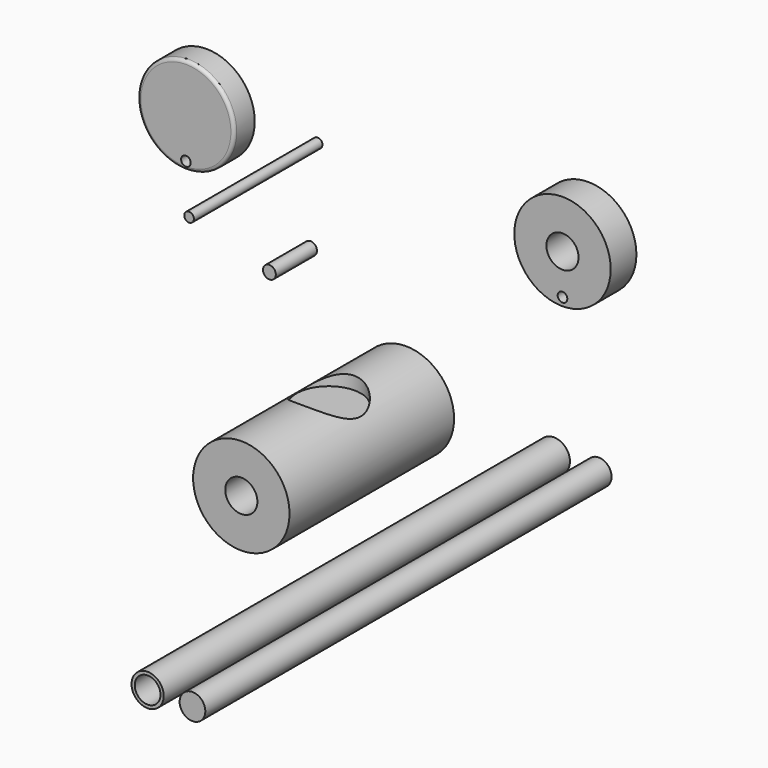
from build123d import *

# Parameters (mm, degrees)
F0_R      = 15
F0_R_2    = 5
F1_DEPTH  = 64
F2_R      = 2
F2_R_2    = 5
F3_DEPTH  = 3
F4_R      = 15
F4_R_2    = 2
F4_R_3    = 5
F5_DEPTH  = 10
F6_R      = 15
F6_R_2    = 1.5
F6_R_3    = 5
F7_DEPTH  = 2
F9_R      = 10
F10_DEPTH = 4
F11_R     = 5
F11_R_2   = 4
F12_DEPTH = 158
F13_R     = 4
F14_DEPTH = 158
F15_R     = 2
F16_DEPTH = 16
F17_R     = 15
F17_R_2   = 1.5
F18_DEPTH = 8
F19_R     = 1.5
F20_DEPTH = 50
F21_R     = 0.99999
F17_R_3   = 5
F22_DEPTH = 10
F23_R     = 5
F24_DEPTH = 5


# Not quite as in the source:
# - a fillet or chamfer is up to 0.001 mm smaller than in the source, because OpenCascade refuses the exact size
# - a feature names something its author has since deleted; it is built from what else it names


with BuildPart() as f1:
    # F0 (on Front) → F1 (new body)
    with BuildSketch(Plane.XZ):
        Circle(F0_R)
        Circle(F0_R_2, mode=Mode.SUBTRACT)
    extrude(amount=F1_DEPTH)

    # F9 (on offset) → F10 (cut)
    with BuildSketch(Plane.XY.offset(15)):
        with Locations((0, -30)):
            Circle(F9_R)
    extrude(amount=-F10_DEPTH, mode=Mode.SUBTRACT)


with BuildPart() as f3:
    # F2 (on Front) → F3 (new body)
    with BuildSketch(Plane.XZ):
        with BuildLine():
            Line((-54.3058665821, 6.5412230759), (-51.4285073808, 3.7625895941))
            ThreePointArc((-51.4285073808, 3.7625895941), (-48.3108465674, 8.5633662497), (-47.2186043859, 14.182465151))
            ThreePointArc((-47.2186043859, 14.182465151), (-67.8377032871, 28.0902229695), (-73.0087013909, 3.7625895941))
            Line((-73.0087013909, 3.7625895941), (-70.1313421896, 6.5412230759))
            ThreePointArc((-70.1313421896, 6.5412230759), (-62.2186043859, 3.182465151), (-54.3058665821, 6.5412230759))
        make_face()
        with Locations((-72.2186043859, 14.182465151)):
            Circle(F2_R, mode=Mode.SUBTRACT)
        with Locations((-62.2186043859, 14.182465151)):
            Circle(F2_R_2, mode=Mode.SUBTRACT)
        with BuildLine():
            ThreePointArc((-54.2186043859, 14.182465151), (-52.2186043859, 16.182465151), (-50.2186043859, 14.182465151))
            ThreePointArc((-50.2186043859, 14.182465151), (-52.2186043859, 12.182465151), (-54.2186043859, 14.182465151))
        make_face(mode=Mode.SUBTRACT)
    extrude(amount=F3_DEPTH)


with BuildPart() as f5:
    # F4 (on Front) → F5 (new body)
    with BuildSketch(Plane.XZ):
        with Locations((-47.7725118399, -37.5088863075)):
            Circle(F4_R)
        with Locations((-57.7725118399, -37.5088863075)):
            Circle(F4_R_2, mode=Mode.SUBTRACT)
        with Locations((-47.7725118399, -37.5088863075)):
            Circle(F4_R_3, mode=Mode.SUBTRACT)
        with Locations((-37.7725118399, -37.5088863075)):
            Circle(F4_R_2, mode=Mode.SUBTRACT)
    extrude(amount=F5_DEPTH)


with BuildPart() as f7:
    # F6 (on Front) → F7 (new body)
    with BuildSketch(Plane.XZ):
        with Locations((12.6999374479, 49.0343069208)):
            Circle(F6_R)
        with Locations((12.6999374479, 36.5343069208)):
            Circle(F6_R_2, mode=Mode.SUBTRACT)
        with Locations((12.6999374479, 49.0343069208)):
            Circle(F6_R_3, mode=Mode.SUBTRACT)
    extrude(amount=F7_DEPTH)


with BuildPart() as f12:
    # F11 (on Front) → F12 (new body)
    with BuildSketch(Plane.XZ):
        with Locations((46.0497015125, 0)):
            Circle(F11_R)
        with Locations((46.0497015125, 0)):
            Circle(F11_R_2, mode=Mode.SUBTRACT)
    extrude(amount=F12_DEPTH)


with BuildPart() as f14:
    # F13 (on Front) → F14 (new body)
    with BuildSketch(Plane.XZ):
        with Locations((60, 0)):
            Circle(F13_R)
    extrude(amount=F14_DEPTH)


with BuildPart() as f16:
    # F15 (on Front) → F16 (new body)
    with BuildSketch(Plane.XZ):
        with Locations((-29.6608433127, 32.0971570909)):
            Circle(F15_R)
    extrude(amount=F16_DEPTH)


with BuildPart() as f18:
    # F17 (on Front) → F18 (new body)
    with BuildSketch(Plane.XZ):
        with Locations((-62.032982707, 61.2359903753)):
            Circle(F17_R)
        with Locations((-62.032982707, 48.7359903753)):
            Circle(F17_R_2, mode=Mode.SUBTRACT)
    extrude(amount=F18_DEPTH)

    # F21 (radius 1 in the source; OpenCascade refuses exactly that, so slightly less here)
    f21_edges = [f18.edges().sort_by_distance(p)[0] for p in [
        (-77.032983, -8, 61.23599),
    ]]
    fillet(f21_edges, radius=F21_R)

    # F23 (on face) → F24 (cut)
    with BuildSketch(Plane(origin=(0, 0, 0), x_dir=(-1, 0, 0), z_dir=(0, 1, 0))):
        with Locations((62.032982707, 61.2359903753)):
            Circle(F23_R)
    extrude(amount=-F24_DEPTH, mode=Mode.SUBTRACT)


with BuildPart() as f20:
    # F19 (on Front) → F20 (new body)
    with BuildSketch(Plane.XZ):
        with Locations((-27.4534914643, 61.705391854)):
            Circle(F19_R)
    extrude(amount=F20_DEPTH)


with BuildPart() as f22:
    # F17 (on Front) → F22 (new body)
    with BuildSketch(Plane.XZ):
        with Locations((56.7282065749, 63.4172449509)):
            Circle(F17_R)
        with Locations((56.7282065749, 50.9172449509)):
            Circle(F17_R_2, mode=Mode.SUBTRACT)
        with Locations((56.7282065749, 63.4172449509)):
            Circle(F17_R_3, mode=Mode.SUBTRACT)
    extrude(amount=F22_DEPTH)


solid = Compound([f1.part, f12.part, f14.part, f16.part, f18.part, f20.part, f22.part])
